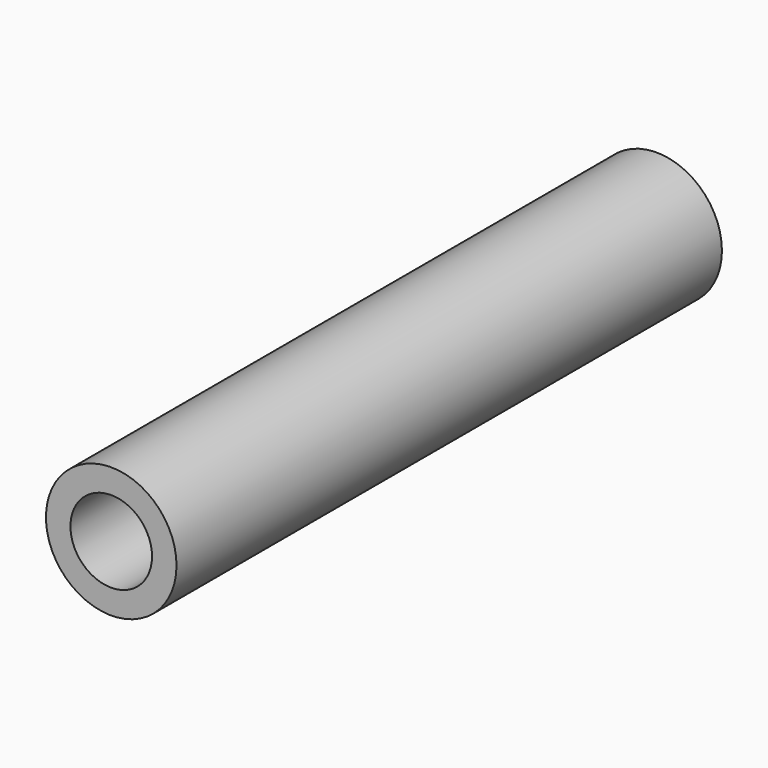
from build123d import *

# Parameters (mm, degrees)
F0_R     = 3.6
F1_DEPTH = 37.6
F2_R     = 2.25
F3_DEPTH = 38.1


# Not quite as in the source:
# - a feature of the source that left no trace in its solid (it failed there, or was rolled back) is left out
# - the program builds the solid bodies; features that only make, move or delete a surface that nothing else refers to are left out


with BuildPart() as f1:
    # F0 (on Front) → F1 (new body)
    with BuildSketch(Plane.XZ):
        Circle(F0_R)
    extrude(amount=F1_DEPTH)

    # F2 (on Front) → F3 (cut)
    with BuildSketch(Plane.XZ):
        Circle(F2_R)
    extrude(amount=F3_DEPTH, mode=Mode.SUBTRACT)


solid = f1.part
